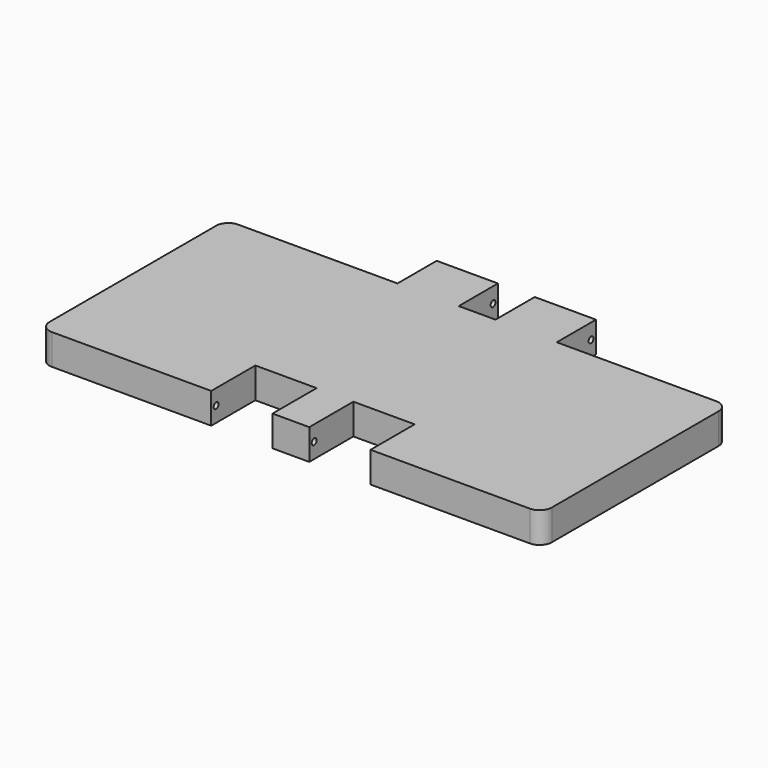
from build123d import *

# Parameters (mm, degrees)
F1_DEPTH  = 5
F2_R      = 0.5
F3_DEPTH  = 2
F4_R      = 0.5
F5_DEPTH  = 5
F6_R      = 0.5
F7_DEPTH  = 2
F8_R      = 0.5
F9_DEPTH  = 5
F10_R     = 0.5
F11_DEPTH = 14.478


with BuildPart() as f1:
    # F0 (on Top) → F1 (new body)
    with BuildSketch(Plane.XY):
        with BuildLine():
            ThreePointArc((-39, 19), (-40.4142135624, 18.4142135624), (-41, 17))
            Line((-41, 17), (-41, -17))
            ThreePointArc((-41, -17), (-40.4142135624, -18.4142135624), (-39, -19))
            Line((-39, -19), (-13, -19))
            Line((-13, -19), (-13, -10))
            Line((-13, -10), (-3, -10))
            Line((-3, -10), (-3, -19))
            Line((-3, -19), (3, -19))
            Line((3, -19), (3, -10))
            Line((3, -10), (13, -10))
            Line((13, -10), (13, -19))
            Line((13, -19), (39, -19))
            ThreePointArc((39, -19), (40.4142135624, -18.4142135624), (41, -17))
            Line((41, -17), (41, 17))
            ThreePointArc((41, 17), (40.4142135624, 18.4142135624), (39, 19))
            Line((39, 19), (13, 19))
            Line((13, 19), (13, 27))
            Line((13, 27), (3, 27))
            Line((3, 27), (3, 19))
            Line((3, 19), (-3, 19))
            Line((-3, 19), (-3, 27))
            Line((-3, 27), (-13, 27))
            Line((-13, 27), (-13, 19))
            Line((-13, 19), (-39, 19))
        make_face()
    extrude(amount=F1_DEPTH)

    # F2 (on face) → F3 (cut)
    with BuildSketch(Plane.YZ.offset(3)):
        with Locations((-18, 2.5)):
            Circle(F2_R)
    extrude(amount=-F3_DEPTH, mode=Mode.SUBTRACT)

    # F4 (on face) → F5 (cut)
    with BuildSketch(Plane(origin=(13, 0, 0), x_dir=(0, -1, 0), z_dir=(-1, 0, 0))):
        with Locations((13, 2.5)):
            Circle(F4_R)
    extrude(amount=-F5_DEPTH, mode=Mode.SUBTRACT)

    # F6 (on face) → F7 (cut)
    with BuildSketch(Plane(origin=(-3, 0, 0), x_dir=(0, -1, 0), z_dir=(-1, 0, 0))):
        with Locations((18, 2.5)):
            Circle(F6_R)
    extrude(amount=-F7_DEPTH, mode=Mode.SUBTRACT)

    # F8 (on face) → F9 (cut)
    with BuildSketch(Plane.YZ.offset(-13)):
        with Locations((-18, 2.5)):
            Circle(F8_R)
    extrude(amount=-F9_DEPTH, mode=Mode.SUBTRACT)

    # F10 (on Right) → F11 (cut, symmetric)
    with BuildSketch(Plane.YZ):
        with Locations((26, 2.5)):
            Circle(F10_R)
    extrude(amount=F11_DEPTH, both=True, mode=Mode.SUBTRACT)


solid = f1.part
